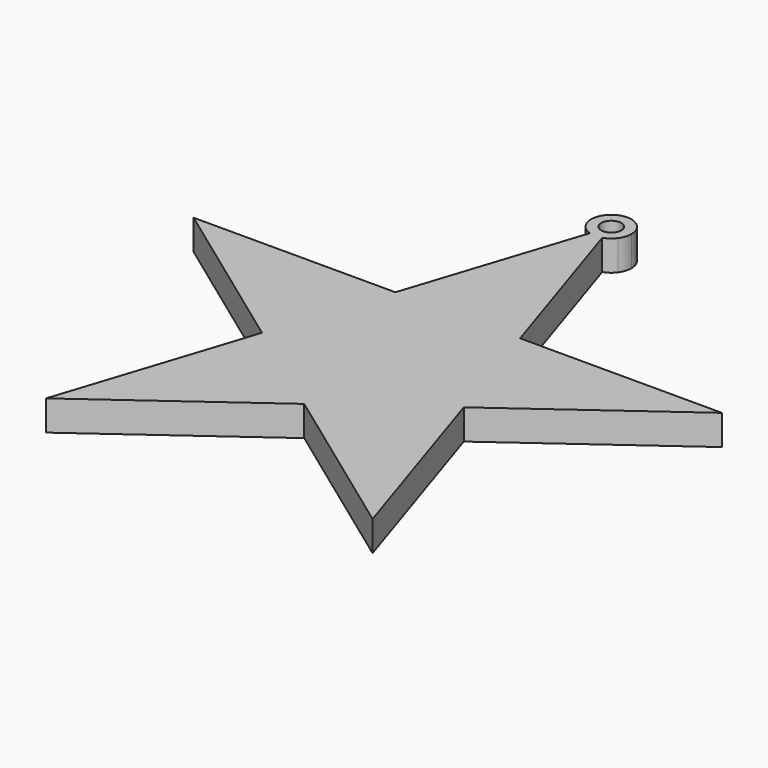
from build123d import *

# Parameters (mm, degrees)
F1_DEPTH = 3


# Not quite as in the source:
# - a feature names something its author has since deleted; it is built from what else it names


with BuildPart() as f1:
    # F0 (on Top) → F1 (new body)
    with BuildSketch(Plane.XY):
        with BuildLine():
            ThreePointArc((0.6180339887, 25.7372071924), (0, 25.639320225), (-0.6180339887, 25.7372071924))
            Line((-0.6180339887, 25.7372071924), (-6.2054140173, 8.5410196625))
            Line((-6.2054140173, 8.5410196625), (-26.286555606, 8.5410196625))
            Line((-26.286555606, 8.5410196625), (-10.0405707943, -3.2623792125))
            Line((-10.0405707943, -3.2623792125), (-16.2459848116, -22.360679775))
            Line((-16.2459848116, -22.360679775), (0, -10.5572809))
            Line((0, -10.5572809), (16.2459848116, -22.360679775))
            Line((16.2459848116, -22.360679775), (10.0405707943, -3.2623792125))
            Line((10.0405707943, -3.2623792125), (26.286555606, 8.5410196625))
            Line((26.286555606, 8.5410196625), (6.2054140173, 8.5410196625))
            Line((6.2054140173, 8.5410196625), (0.6180339887, 25.7372071924))
        make_face()
        with BuildLine():
            ThreePointArc((0.3090169944, 26.6882637087), (0, 26.639320225), (-0.3090169944, 26.6882637087))
            Line((-0.3090169944, 26.6882637087), (-0.6180339887, 25.7372071924))
            ThreePointArc((-0.6180339887, 25.7372071924), (0, 25.639320225), (0.6180339887, 25.7372071924))
            Line((0.6180339887, 25.7372071924), (0.3090169944, 26.6882637087))
        make_face()
        with BuildLine():
            Line((1.6180339887, 26.4637497204), (0.8090169944, 27.0515349727))
            ThreePointArc((0.8090169944, 27.0515349727), (0.5877852523, 26.8303032306), (0.3090169944, 26.6882637087))
            Line((0.3090169944, 26.6882637087), (0.6180339887, 25.7372071924))
            ThreePointArc((0.6180339887, 25.7372071924), (1.1755705046, 26.0212862363), (1.6180339887, 26.4637497204))
        make_face()
        with BuildLine():
            ThreePointArc((1, 27.639320225), (0.9510565163, 27.3303032306), (0.8090169944, 27.0515349727))
            Line((0.8090169944, 27.0515349727), (1.6180339887, 26.4637497204))
            ThreePointArc((1.6180339887, 26.4637497204), (1.9021130326, 27.0212862363), (2, 27.639320225))
            ThreePointArc((2, 27.639320225), (-0.6180339887, 29.5414332576), (-1.6180339887, 26.4637497204))
            Line((-1.6180339887, 26.4637497204), (-0.8090169944, 27.0515349727))
            ThreePointArc((-0.8090169944, 27.0515349727), (-0.3090169944, 28.5903767413), (1, 27.639320225))
        make_face()
        with BuildLine():
            ThreePointArc((-0.3090169944, 26.6882637087), (-0.5877852523, 26.8303032306), (-0.8090169944, 27.0515349727))
            Line((-0.8090169944, 27.0515349727), (-1.6180339887, 26.4637497204))
            ThreePointArc((-1.6180339887, 26.4637497204), (-1.1755705046, 26.0212862363), (-0.6180339887, 25.7372071924))
            Line((-0.6180339887, 25.7372071924), (-0.3090169944, 26.6882637087))
        make_face()
    extrude(amount=F1_DEPTH)


solid = f1.part
